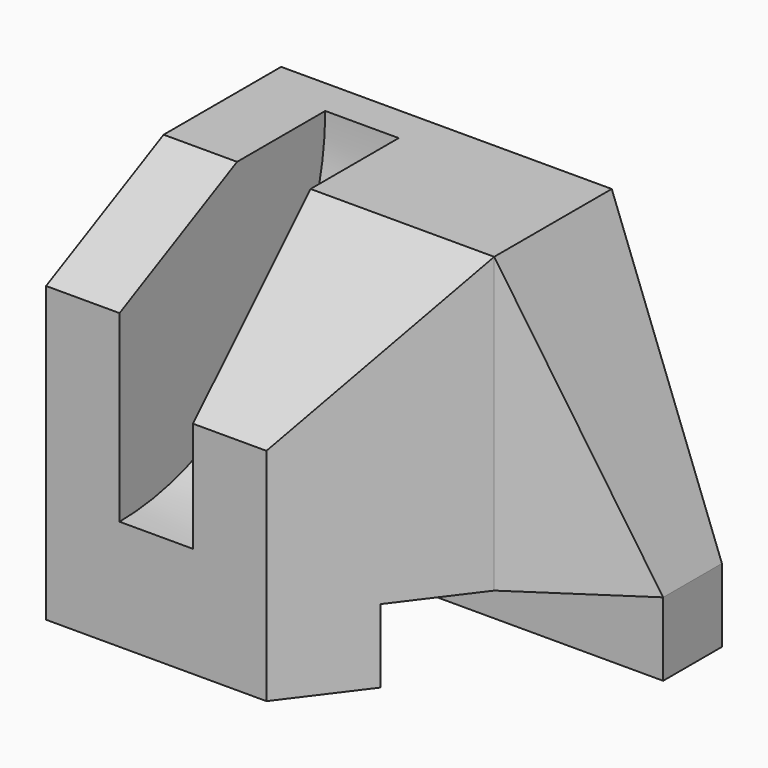
from build123d import *

# Parameters (mm, degrees)
F0_W      = 60
F0_H      = 40
F1_DEPTH  = 50
F2_W      = 20
F2_H      = 10
F3_DEPTH  = 60.001
F5_DEPTH  = 50.001
F9_W      = 10
F9_H      = 35
F10_DEPTH = 35
F11_R     = 34.99999
F12_W     = 10
F12_H     = 20
F16_DEPTH = 40.001


# Not quite as in the source:
# - a fillet or chamfer is up to 0.001 mm smaller than in the source, because OpenCascade refuses the exact size


with BuildPart() as f1:
    # F0 (on Top) → F1 (new body)
    with BuildSketch(Plane.XY):
        with Locations((30, 20)):
            Rectangle(F0_W, F0_H)
    extrude(amount=F1_DEPTH)

    # F2 (on face) → F3 (cut, through all)
    with BuildSketch(Plane.YZ.offset(60)):
        with Locations((20, 5)):
            Rectangle(F2_W, F2_H)
    extrude(amount=-F3_DEPTH, mode=Mode.SUBTRACT)

    # F4 (on face) → F5 (cut, through all)
    with BuildSketch(Plane.XY.offset(50)):
        Polygon((45, 20), (30, 0), (60, 0), (60, 10), (60, 30), align=None)
    extrude(amount=-F5_DEPTH, mode=Mode.SUBTRACT)

    # F8: sweep along a path in F7
    with BuildLine(Plane.YZ.offset(60)) as f8_path:
        Line((20, 50), (0, 30))
    # F6 (on face) → F8 (sweep, cut)
    with BuildSketch(Plane.XY.offset(50)):
        Polygon((30, 0), (45, 20), (20, 20), (20, 0), align=None)
    sweep(path=f8_path.line, mode=Mode.SUBTRACT)

    # F9 (on face) → F10 (cut)
    with BuildSketch(Plane.XY.offset(50)):
        with Locations((15, 17.5)):
            Rectangle(F9_W, F9_H)
    extrude(amount=-F10_DEPTH, mode=Mode.SUBTRACT)

    # F11 (radius 35 in the source; OpenCascade refuses exactly that, so slightly less here)
    f11_edges = [f1.edges().sort_by_distance(p)[0] for p in [
        (15, 35, 15),
    ]]
    fillet(f11_edges, radius=F11_R)

    # F14: sweep along a path in F13
    with BuildLine(Plane(origin=(0, 0, 0), x_dir=(0, -1, 0), z_dir=(-1, 0, 0))) as f14_path:
        Line((0, 40), (-20, 50))
    # F12 (on face) → F14 (sweep, cut)
    with BuildSketch(Plane.XY.offset(50)):
        with Locations((5, 10)):
            Rectangle(F12_W, F12_H)
    sweep(path=f14_path.line, mode=Mode.SUBTRACT)

    # F15 (on face) → F16 (cut, through all)
    with BuildSketch(Plane(origin=(0, 40, 0), x_dir=(-1, 0, 0), z_dir=(0, 1, 0))):
        Polygon((-60, 10), (-45, 50), (-60, 50), align=None)
    extrude(amount=-F16_DEPTH, mode=Mode.SUBTRACT)


solid = f1.part
